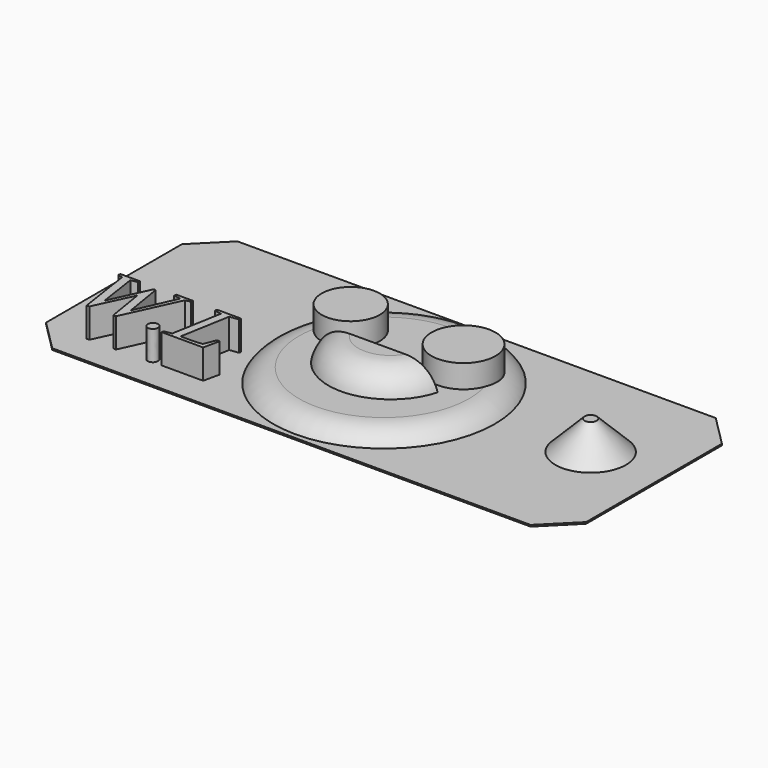
from build123d import *

# Parameters (mm, degrees)
F1_R          = 18.3919113819
F2_DEPTH      = 2.54
F3_R          = 4.7807571244
F4_DEPTH      = 3.81
F5_R          = 5.2628283108
F6_DEPTH      = 3.81
F8_DEPTH      = 3.81
F11_R         = 6.0721906368
F12_DEPTH     = 5.08
F14_TEXT_SIZE = 14.2415590946
F15_DEPTH     = 5.08
F17_S5_R      = 4.7807571244
F17_T6_DEPTH  = 31
F17_S7_R      = 5.2628283108
F17_T8_DEPTH  = 31
F17_T12_ANGLE = 286.6836927305
F18_SIZE      = 5.07999
F0_W          = 88.9
F0_H          = 38.1
F19_DEPTH     = 0.254
F20_SIZE      = 5.08


# Not quite as in the source:
# - a fillet or chamfer that OpenCascade refuses, or shapes differently, is made with other operations: its cross-section is extruded or revolved along the edge and cut away or added
# - a fillet or chamfer is up to 0.001 mm smaller than in the source, because OpenCascade refuses the exact size
# - a feature of the source that left no trace in its solid (it failed there, or was rolled back) is left out
# - the program builds the solid bodies; features that only make, move or delete a surface that nothing else refers to are left out
# - Text() gives the source's letters only with a copy of the font that has no kerning and outlines rounded to 1/6400 em; it was checked with that copy


with BuildPart() as f2:
    # F1 (on face) → F2 (new body)
    with BuildSketch(Plane.XY):
        Circle(F1_R)
    extrude(amount=F2_DEPTH)

    # F3 (on face) → F4 (join)
    with BuildSketch(Plane.XY.offset(2.54)):
        with Locations((-9.7671682015, 5.3561157547)):
            Circle(F3_R)
    extrude(amount=F4_DEPTH)

    # F5 (on face) → F6 (join)
    with BuildSketch(Plane.XY.offset(2.54)):
        with Locations((8.5303336382, 5.6983716786)):
            Circle(F5_R)
    extrude(amount=F6_DEPTH)

    # F7 (on face) → F8 (join)
    with BuildSketch(Plane.XY.offset(2.54)):
        with BuildLine():
            Line((9.7374357283, -1.1452846229), (-10.0281173363, -1.1696107686))
            ThreePointArc((-10.0281173363, -1.1696107686), (-0.1360832097, -8.6794560846), (9.7374357283, -1.1452846229))
        make_face()
    extrude(amount=F8_DEPTH)

    # F17: fillet of radius 5.08 on 2 edges, made by hand


with BuildPart() as f12:
    # F11 (on face) → F12 (new body)
    with BuildSketch(Plane.XY):
        with Locations((32.6933060888, 1.654658673)):
            Circle(F11_R)
    extrude(amount=F12_DEPTH)

    # F18 (size 5.08 in the source; OpenCascade refuses exactly that, so slightly less here)
    f18_edges = [f12.edges().sort_by_distance(p)[0] for p in [
        (26.621115, 1.654659, 5.08),
    ]]
    chamfer(f18_edges, length=F18_SIZE)


with BuildPart() as f15:
    # F14 (on face) → F15 (new body)
    with BuildSketch(Plane.XY):
        with Locations((-40.6434871256, -14.0083692968)):
            Text('W.L', F14_TEXT_SIZE, font='Tinos', font_style=FontStyle.ITALIC, text_align=(TextAlign.LEFT, TextAlign.BOTTOM))
    extrude(amount=F15_DEPTH)


with BuildPart() as f17_tool2:
    # F17_s3 → F17_t4 (revolve)
    with BuildSketch(Plane.XZ):
        with BuildLine():
            ThreePointArc((18.3919113819, 0), (16.5325023307, 1.8594090512), (13.9925023307, 2.54))
            Line((13.9925023307, 2.54), (18.3919113819, 2.54))
            Line((18.3919113819, 2.54), (18.3919113819, 0))
        make_face()
    revolve(axis=Axis((0, 0, 2.54), (0, 0, 1)))

    # F17_s5 → F17_t6 (cut, symmetric)
    with BuildSketch(Plane.XY):
        with Locations((-9.7671682015, 5.3561157547)):
            Circle(F17_S5_R)
    extrude(amount=F17_T6_DEPTH, both=True, mode=Mode.SUBTRACT)

    # F17_s7 → F17_t8 (cut, symmetric)
    with BuildSketch(Plane.XY):
        with Locations((8.5303336382, 5.6983716786)):
            Circle(F17_S7_R)
    extrude(amount=F17_T8_DEPTH, both=True, mode=Mode.SUBTRACT)


with BuildPart() as f2_1:
    add(f2.part)

    # F17_t1: cut F17_tool2
    add(f17_tool2.part, mode=Mode.SUBTRACT)


with BuildPart() as f17_tool10:
    # F17_s11 → F17_t12 (revolve)
    with BuildSketch(Plane(origin=(0.6587988504, 0.4915665164, 0), x_dir=(0, 0, 1), z_dir=(0.8014765061, 0.5980262622, 0))):
        with BuildLine():
            ThreePointArc((2.54, -11.6035225538), (5.2860926284, -9.7956856774), (6.35, -6.6848337041))
            Line((6.35, -6.6848337041), (6.35, -11.6035225538))
            Line((6.35, -11.6035225538), (2.54, -11.6035225538))
        make_face()
    revolve(axis=Axis((-0.148702222, 1.573781762, 6.35), (0, 0, 1)), revolution_arc=F17_T12_ANGLE)

    split(bisect_by=Plane(origin=(0.0014242884, -1.1572670669, 0), x_dir=(0, 0, 1), z_dir=(0.0012307334, -0.9999992426, 0)), keep=Keep.TOP)


with BuildPart() as f2_2:
    add(f2_1.part)

    # F17_t9: cut F17_tool10
    add(f17_tool10.part, mode=Mode.SUBTRACT)


with BuildPart() as f19:
    # F0 (on Top) → F19 (new body)
    with BuildSketch(Plane.XY):
        Rectangle(F0_W, F0_H)
    extrude(amount=F19_DEPTH)

    # F20
    f20_edges = [f19.edges().sort_by_distance(p)[0] for p in [
        (44.45, -19.05, 0.127),
        (44.45, 19.05, 0.127),
        (-44.45, -19.05, 0.127),
        (-44.45, 19.05, 0.127),
    ]]
    chamfer(f20_edges, length=F20_SIZE)


solid = Compound([f12.part, f15.part, f2_2.part, f19.part])
